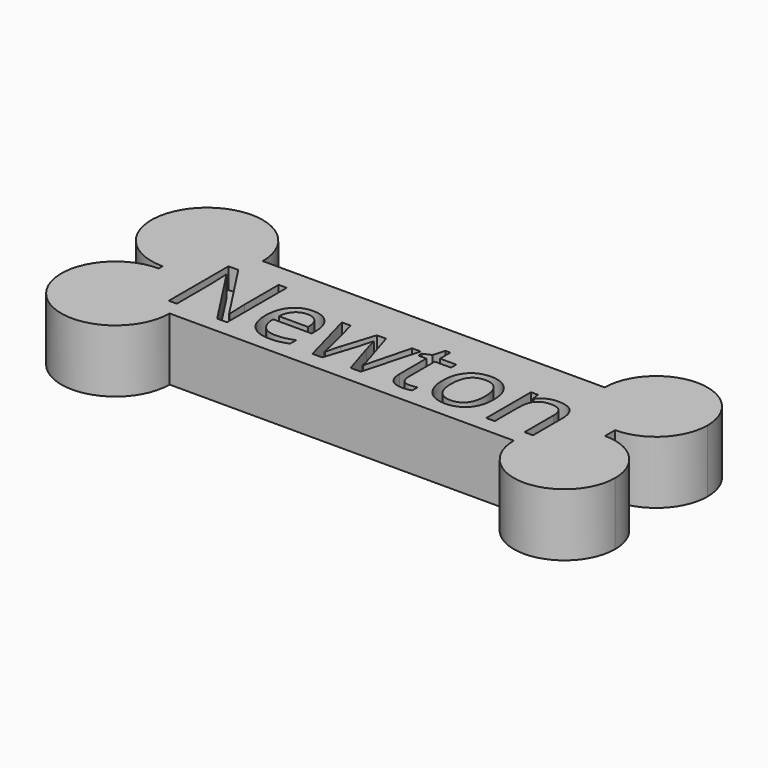
from build123d import *

# Parameters (mm, degrees)
F1_DEPTH     = 5.334
F2_TEXT_SIZE = 8.8959605718
F3_DEPTH     = 1.778


# Not quite as in the source:
# - Text() gives the source's letters only with a copy of the font that has no kerning and outlines rounded to 1/6400 em; it was checked with that copy


with BuildPart() as f1:
    # F0 (on Top) → F1 (new body)
    with BuildSketch(Plane.XY):
        with BuildLine():
            ThreePointArc((-38.2284894586, -4.7386302631), (-34.877771866, -3.3507175926), (-33.4898591954, 0))
            Line((-33.4898591954, 0), (-38.2284894586, 0))
            Line((-38.2284894586, 0), (-38.2284894586, -4.7386302631))
        make_face()
        with BuildLine():
            Line((-38.2284894586, 0), (-33.4898591954, 0))
            ThreePointArc((-33.4898591954, 0), (-41.5792070511, 3.3507175926), (-38.2284894586, -4.7386302631))
            Line((-38.2284894586, -4.7386302631), (-38.2284894586, 0))
        make_face()
        with BuildLine():
            Line((-4.3768007177, 0), (-33.4898591954, 0))
            ThreePointArc((-33.4898591954, 0), (-34.877771866, -3.3507175926), (-38.2284894586, -4.7386302631))
            Line((-38.2284894586, -4.7386302631), (-38.2284894586, -5.145930946))
            ThreePointArc((-38.2284894586, -5.145930946), (-34.9696202421, -6.4957987734), (-33.6197524146, -9.7546679899))
            Line((-33.6197524146, -9.7546679899), (-4.3096074711, -9.7546679899))
            ThreePointArc((-4.3096074711, -9.7546679899), (-3.047352667, -6.7073153229), (0, -5.4450605188))
            Line((0, -5.4450605188), (0, -4.3768007177))
            ThreePointArc((0, -4.3768007177), (-3.0948654674, -3.0948654674), (-4.3768007177, 0))
        make_face()
        with BuildLine():
            ThreePointArc((4.3768007177, 0), (0, 4.3768007177), (-4.3768007177, 0))
            Line((-4.3768007177, 0), (0, 0))
            Line((0, 0), (0, -4.3768007177))
            ThreePointArc((0, -4.3768007177), (3.0948654674, -3.0948654674), (4.3768007177, 0))
        make_face()
        with BuildLine():
            Line((0, 0), (-4.3768007177, 0))
            ThreePointArc((-4.3768007177, 0), (-3.0948654674, -3.0948654674), (0, -4.3768007177))
            Line((0, -4.3768007177), (0, 0))
        make_face()
        with BuildLine():
            ThreePointArc((-33.6197524146, -9.7546679899), (-34.9696202421, -6.4957987734), (-38.2284894586, -5.145930946))
            Line((-38.2284894586, -5.145930946), (-38.2284894586, -9.7546679899))
            Line((-38.2284894586, -9.7546679899), (-33.6197524146, -9.7546679899))
        make_face()
        with BuildLine():
            Line((-38.2284894586, -9.7546679899), (-38.2284894586, -5.145930946))
            ThreePointArc((-38.2284894586, -5.145930946), (-41.487358675, -13.0135372064), (-33.6197524146, -9.7546679899))
            Line((-33.6197524146, -9.7546679899), (-38.2284894586, -9.7546679899))
        make_face()
        with BuildLine():
            ThreePointArc((4.3096074711, -9.7546679899), (3.047352667, -6.7073153229), (0, -5.4450605188))
            Line((0, -5.4450605188), (0, -9.7546679899))
            Line((0, -9.7546679899), (-4.3096074711, -9.7546679899))
            ThreePointArc((-4.3096074711, -9.7546679899), (0, -14.064275461), (4.3096074711, -9.7546679899))
        make_face()
        with BuildLine():
            Line((0, -9.7546679899), (0, -5.4450605188))
            ThreePointArc((0, -5.4450605188), (-3.047352667, -6.7073153229), (-4.3096074711, -9.7546679899))
            Line((-4.3096074711, -9.7546679899), (0, -9.7546679899))
        make_face()
    extrude(amount=F1_DEPTH)

    # F2 (on face) → F3 (cut)
    with BuildSketch(Plane.XY.offset(5.334)):
        with Locations((-35.6715336093, -8.3600520156)):
            Text('Newton', F2_TEXT_SIZE, font='Open Sans', text_align=(TextAlign.LEFT, TextAlign.BOTTOM))
    extrude(amount=-F3_DEPTH, mode=Mode.SUBTRACT)


solid = f1.part
